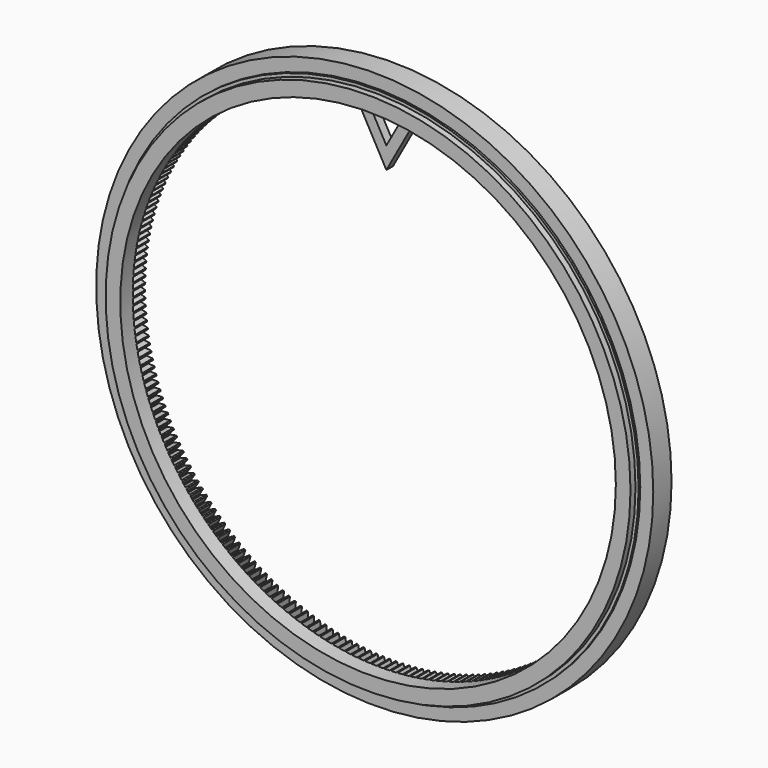
from build123d import *

# Parameters (mm, degrees)
F0_R     = 67
F0_R_2   = 59.6
F1_DEPTH = 3.75
F2_R     = 63.875
F2_R_2   = 63.125
F3_DEPTH = 1.5
F4_DEPTH = 2
F6_DEPTH = 6.5
F7_COUNT = 240
F9_DEPTH = 2


with BuildPart() as f1:
    # F0 (on Front) → F1 (new body, symmetric)
    with BuildSketch(Plane.XZ):
        Circle(F0_R)
        Circle(F0_R_2, mode=Mode.SUBTRACT)
    extrude(amount=F1_DEPTH, both=True)

    # F2 (on face) → F3 (cut)
    with BuildSketch(Plane.XZ.offset(3.75)):
        Circle(F2_R)
        Circle(F2_R_2, mode=Mode.SUBTRACT)
    extrude(amount=-F3_DEPTH, mode=Mode.SUBTRACT)

    # F4 (cut): a face of the model
    f4_faces = [f1.faces().sort_by_distance(p)[0] for p in [
        (-65.1049538264, -3.75, 0),
    ]]
    extrude(f4_faces, amount=-F4_DEPTH, mode=Mode.SUBTRACT)

    # F5 (on Front) → F6 (cut)
    with BuildSketch(Plane.XZ):
        Polygon((61, -0.15), (61, 0.15), (59.4, 0.675), (59.4, -0.675), align=None)
    f6 = extrude(amount=-F6_DEPTH, mode=Mode.SUBTRACT)

    # F7: F6 ×240 about axis
    f7_axis = Axis((0, -3.75, 0), (0, -1, 0))
    for i in range(1, F7_COUNT):
        add(f6.rotate(f7_axis, i * 360 / F7_COUNT), mode=Mode.SUBTRACT)

    # F8 (on face) → F9 (join)
    with BuildSketch(Plane(origin=(0, 3.75, 0), x_dir=(-1, 0, 0), z_dir=(0, 1, 0))):
        with BuildLine():
            Line((0, 45), (8.2146170005, 59.9074033502))
            Line((8.2146170005, 59.9074033502), (8.1108144546, 60.458557615))
            Line((8.1108144546, 60.458557615), (7.8133809962, 60.4977154726))
            Line((7.8133809962, 60.4977154726), (7.1737744537, 59.1666879256))
            ThreePointArc((7.1737744537, 59.1666879256), (7.0052288885, 59.1868800345), (6.8366264964, 59.206592016))
            Line((6.8366264964, 59.206592016), (6.5254145436, 60.650156348))
            Line((6.5254145436, 60.650156348), (6.227057975, 60.681514887))
            Line((6.227057975, 60.681514887), (5.622512849, 59.3342005024))
            ThreePointArc((5.622512849, 59.3342005024), (5.4534964723, 59.3499736834), (5.2844358566, 59.365265414))
            Line((5.2844358566, 59.365265414), (4.9355424395, 60.8001884934))
            Line((4.9355424395, 60.8001884934), (4.6364672393, 60.8237262221))
            Line((4.6364672393, 60.8237262221), (4.0673978548, 59.461048382))
            ThreePointArc((4.0673978548, 59.461048382), (3.8980265021, 59.472391825), (3.7286235284, 59.4832528245))
            Line((3.7286235284, 59.4832528245), (3.342287761, 60.9085512266))
            Line((3.342287761, 60.9085512266), (3.0426989006, 60.9242520135))
            Line((3.0426989006, 60.9242520135), (2.5094952693, 59.5471446292))
            ThreePointArc((2.5094952693, 59.5471446292), (2.3398850192, 59.5540505599), (2.1702557879, 59.5604733847))
            Line((2.1702557879, 59.5604733847), (1.7467424455, 60.9751702813))
            Line((1.7467424455, 60.9751702813), (1.446845248, 60.9830233658))
            Line((1.446845248, 60.9830233658), (0.9498728011, 59.5924302379))
            ThreePointArc((0.9498728011, 59.5924302379), (0.7801398961, 59.5948939234), (0.6104006624, 59.5968741716))
            Line((0.6104006624, 59.5968741716), (0.15, 61))
            Line((0.15, 61), (-0.15, 61))
            Line((-0.15, 61), (-0.6104006624, 59.5968741716))
            ThreePointArc((-0.6104006624, 59.5968741716), (-0.7801398961, 59.5948939234), (-0.9498728011, 59.5924302379))
            Line((-0.9498728011, 59.5924302379), (-1.446845248, 60.9830233658))
            Line((-1.446845248, 60.9830233658), (-1.7467424455, 60.9751702813))
            Line((-1.7467424455, 60.9751702813), (-2.1702557879, 59.5604733847))
            ThreePointArc((-2.1702557879, 59.5604733847), (-2.3398850192, 59.5540505599), (-2.5094952693, 59.5471446292))
            Line((-2.5094952693, 59.5471446292), (-3.0426989006, 60.9242520135))
            Line((-3.0426989006, 60.9242520135), (-3.342287761, 60.9085512266))
            Line((-3.342287761, 60.9085512266), (-3.7286235284, 59.4832528245))
            ThreePointArc((-3.7286235284, 59.4832528245), (-3.8980265021, 59.472391825), (-4.0673978548, 59.461048382))
            Line((-4.0673978548, 59.461048382), (-4.6364672393, 60.8237262221))
            Line((-4.6364672393, 60.8237262221), (-4.9355424395, 60.8001884934))
            Line((-4.9355424395, 60.8001884934), (-5.2844358566, 59.365265414))
            ThreePointArc((-5.2844358566, 59.365265414), (-5.4534964723, 59.3499736834), (-5.622512849, 59.3342005024))
            Line((-5.622512849, 59.3342005024), (-6.227057975, 60.681514887))
            Line((-6.227057975, 60.681514887), (-6.5254145436, 60.650156348))
            Line((-6.5254145436, 60.650156348), (-6.8366264964, 59.206592016))
            ThreePointArc((-6.8366264964, 59.206592016), (-7.0052288885, 59.1868800345), (-7.1737744537, 59.1666879256))
            Line((-7.1737744537, 59.1666879256), (-7.8133809962, 60.4977154726))
            Line((-7.8133809962, 60.4977154726), (-8.1108144546, 60.458557615))
            Line((-8.1108144546, 60.458557615), (-8.2146170005, 59.9074033502))
            Line((-8.2146170005, 59.9074033502), (0, 45))
        make_face()
        Polygon((0.1226131216, 57.9978654854), (4.2828298312, 57.9522886108), (0, 50.1800611569), (-4.2828298312, 57.9522886108), (-0.1226131216, 57.9978654854), align=None, mode=Mode.SUBTRACT)
    extrude(amount=-F9_DEPTH)


solid = f1.part
